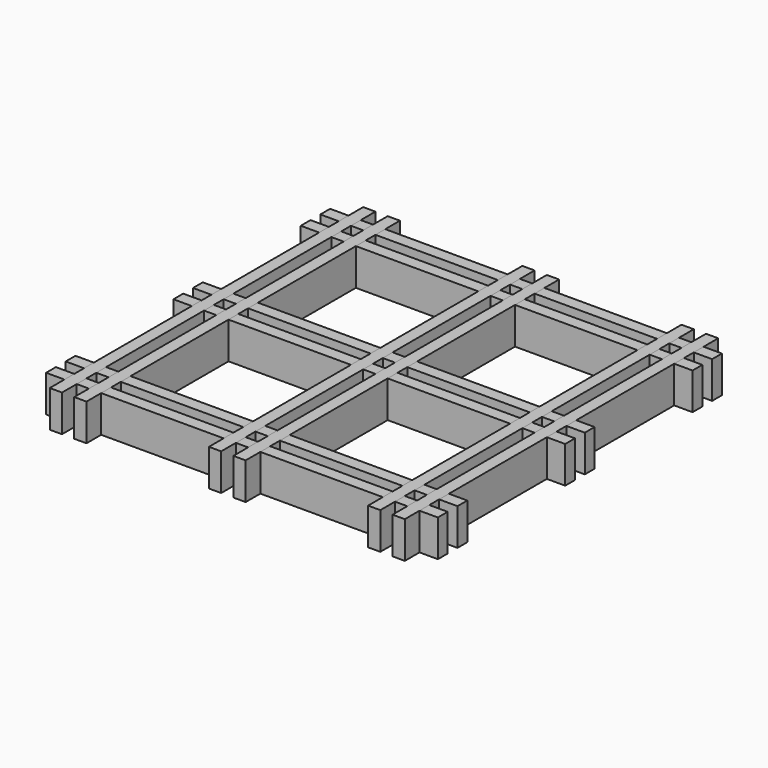
from build123d import *

# Parameters (mm, degrees)
F0_W     = 3.175
F0_H     = 101.6
F1_DEPTH = 9.525
F2_W     = 3.175
F2_H     = 4.7625
F3_DEPTH = 92.076
F4_W     = 101.6
F4_H     = 3.175
F5_DEPTH = 4.7625
F6_W     = 3.175
F6_H     = 3.175
F6_W_2   = 31.75
F6_W_3   = 4.7625
F7_DEPTH = 4.7625


with BuildPart() as f1:
    # F0 (on Top) → F1 (new body)
    with BuildSketch(Plane.XY):
        with Locations((1.5875, -50.8)):
            Rectangle(F0_W, F0_H)
    extrude(amount=F1_DEPTH)


with BuildPart() as f1b:
    # F0 (on Top) → F1, piece 2 (new body)
    with BuildSketch(Plane.XY):
        with Locations((7.9375, -50.8)):
            Rectangle(F0_W, F0_H)
    extrude(amount=F1_DEPTH)


with BuildPart() as f1c:
    # F0 (on Top) → F1, piece 3 (new body)
    with BuildSketch(Plane.XY):
        with Locations((42.8625, -50.8)):
            Rectangle(F0_W, F0_H)
    extrude(amount=F1_DEPTH)


with BuildPart() as f1d:
    # F0 (on Top) → F1, piece 4 (new body)
    with BuildSketch(Plane.XY):
        with Locations((49.2125, -50.8)):
            Rectangle(F0_W, F0_H)
    extrude(amount=F1_DEPTH)


with BuildPart() as f1e:
    # F0 (on Top) → F1, piece 5 (new body)
    with BuildSketch(Plane.XY):
        with Locations((84.1375, -50.8)):
            Rectangle(F0_W, F0_H)
    extrude(amount=F1_DEPTH)


with BuildPart() as f1f:
    # F0 (on Top) → F1, piece 6 (new body)
    with BuildSketch(Plane.XY):
        with Locations((90.4875, -50.8)):
            Rectangle(F0_W, F0_H)
    extrude(amount=F1_DEPTH)


with BuildPart() as f3_tool:
    # F2 (on face) → F3 (new body, through all)
    with BuildSketch(Plane.YZ.offset(92.075)):
        with Locations((-95.25, 2.38125)):
            Rectangle(F2_W, F2_H)
        with Locations((-47.625, 2.38125)):
            Rectangle(F2_W, F2_H)
        with Locations((-53.975, 2.38125)):
            Rectangle(F2_W, F2_H)
        with Locations((-6.35, 2.38125)):
            Rectangle(F2_W, F2_H)
        with Locations((-12.7, 2.38125)):
            Rectangle(F2_W, F2_H)
        with Locations((-88.9, 2.38125)):
            Rectangle(F2_W, F2_H)
    extrude(amount=-F3_DEPTH)


with BuildPart() as f1_1:
    add(f1.part)

    # F3: cut by f3_tool
    add(f3_tool.part, mode=Mode.SUBTRACT)


with BuildPart() as f1b_1:
    add(f1b.part)

    # F3: cut by f3_tool
    add(f3_tool.part, mode=Mode.SUBTRACT)


with BuildPart() as f1c_1:
    add(f1c.part)

    # F3: cut by f3_tool
    add(f3_tool.part, mode=Mode.SUBTRACT)


with BuildPart() as f1d_1:
    add(f1d.part)

    # F3: cut by f3_tool
    add(f3_tool.part, mode=Mode.SUBTRACT)


with BuildPart() as f1e_1:
    add(f1e.part)

    # F3: cut by f3_tool
    add(f3_tool.part, mode=Mode.SUBTRACT)


with BuildPart() as f1f_1:
    add(f1f.part)

    # F3: cut by f3_tool
    add(f3_tool.part, mode=Mode.SUBTRACT)


with BuildPart() as f5:
    # F4 (on Top) → F5 (new body, through all)
    with BuildSketch(Plane.XY):
        with Locations((46.0375, -6.35)):
            Rectangle(F4_W, F4_H)
    extrude(amount=F5_DEPTH)

    # F6 (on face) → F7, piece 6 (join, through all)
    with BuildSketch(Plane.XY.offset(4.7625)):
        with Locations((4.7625, -6.35)):
            Rectangle(F6_W, F6_H)
        with Locations((25.4, -6.35)):
            Rectangle(F6_W_2, F6_H)
        with Locations((94.45625, -6.35)):
            Rectangle(F6_W_3, F6_H)
        with Locations((-2.38125, -6.35)):
            Rectangle(F6_W_3, F6_H)
        with Locations((46.0375, -6.35)):
            Rectangle(F6_W, F6_H)
        with Locations((87.3125, -6.35)):
            Rectangle(F6_W, F6_H)
        with Locations((66.675, -6.35)):
            Rectangle(F6_W_2, F6_H)
    extrude(amount=F7_DEPTH)


with BuildPart() as f5b:
    # F4 (on Top) → F5, piece 2 (new body, through all)
    with BuildSketch(Plane.XY):
        with Locations((46.0375, -12.7)):
            Rectangle(F4_W, F4_H)
    extrude(amount=F5_DEPTH)

    # F6 (on face) → F7, piece 5 (join, through all)
    with BuildSketch(Plane.XY.offset(4.7625)):
        with Locations((4.7625, -12.7)):
            Rectangle(F6_W, F6_H)
        with Locations((25.4, -12.7)):
            Rectangle(F6_W_2, F6_H)
        with Locations((94.45625, -12.7)):
            Rectangle(F6_W_3, F6_H)
        with Locations((-2.38125, -12.7)):
            Rectangle(F6_W_3, F6_H)
        with Locations((46.0375, -12.7)):
            Rectangle(F6_W, F6_H)
        with Locations((87.3125, -12.7)):
            Rectangle(F6_W, F6_H)
        with Locations((66.675, -12.7)):
            Rectangle(F6_W_2, F6_H)
    extrude(amount=F7_DEPTH)


with BuildPart() as f5c:
    # F4 (on Top) → F5, piece 3 (new body, through all)
    with BuildSketch(Plane.XY):
        with Locations((46.0375, -95.25)):
            Rectangle(F4_W, F4_H)
    extrude(amount=F5_DEPTH)

    # F6 (on face) → F7 (join, through all)
    with BuildSketch(Plane.XY.offset(4.7625)):
        with Locations((4.7625, -95.25)):
            Rectangle(F6_W, F6_H)
        with Locations((25.4, -95.25)):
            Rectangle(F6_W_2, F6_H)
        with Locations((94.45625, -95.25)):
            Rectangle(F6_W_3, F6_H)
        with Locations((-2.38125, -95.25)):
            Rectangle(F6_W_3, F6_H)
        with Locations((46.0375, -95.25)):
            Rectangle(F6_W, F6_H)
        with Locations((87.3125, -95.25)):
            Rectangle(F6_W, F6_H)
        with Locations((66.675, -95.25)):
            Rectangle(F6_W_2, F6_H)
    extrude(amount=F7_DEPTH)


with BuildPart() as f5d:
    # F4 (on Top) → F5, piece 4 (new body, through all)
    with BuildSketch(Plane.XY):
        with Locations((46.0375, -47.625)):
            Rectangle(F4_W, F4_H)
    extrude(amount=F5_DEPTH)

    # F6 (on face) → F7, piece 4 (join, through all)
    with BuildSketch(Plane.XY.offset(4.7625)):
        with Locations((-2.38125, -47.625)):
            Rectangle(F6_W_3, F6_H)
        with Locations((4.7625, -47.625)):
            Rectangle(F6_W, F6_H)
        with Locations((25.4, -47.625)):
            Rectangle(F6_W_2, F6_H)
        with Locations((46.0375, -47.625)):
            Rectangle(F6_W, F6_H)
        with Locations((94.45625, -47.625)):
            Rectangle(F6_W_3, F6_H)
        with Locations((87.3125, -47.625)):
            Rectangle(F6_W, F6_H)
        with Locations((66.675, -47.625)):
            Rectangle(F6_W_2, F6_H)
    extrude(amount=F7_DEPTH)


with BuildPart() as f5e:
    # F4 (on Top) → F5, piece 5 (new body, through all)
    with BuildSketch(Plane.XY):
        with Locations((46.0375, -53.975)):
            Rectangle(F4_W, F4_H)
    extrude(amount=F5_DEPTH)

    # F6 (on face) → F7, piece 3 (join, through all)
    with BuildSketch(Plane.XY.offset(4.7625)):
        with Locations((-2.38125, -53.975)):
            Rectangle(F6_W_3, F6_H)
        with Locations((4.7625, -53.975)):
            Rectangle(F6_W, F6_H)
        with Locations((25.4, -53.975)):
            Rectangle(F6_W_2, F6_H)
        with Locations((46.0375, -53.975)):
            Rectangle(F6_W, F6_H)
        with Locations((87.3125, -53.975)):
            Rectangle(F6_W, F6_H)
        with Locations((94.45625, -53.975)):
            Rectangle(F6_W_3, F6_H)
        with Locations((66.675, -53.975)):
            Rectangle(F6_W_2, F6_H)
    extrude(amount=F7_DEPTH)


with BuildPart() as f5f:
    # F4 (on Top) → F5, piece 6 (new body, through all)
    with BuildSketch(Plane.XY):
        with Locations((46.0375, -88.9)):
            Rectangle(F4_W, F4_H)
    extrude(amount=F5_DEPTH)

    # F6 (on face) → F7, piece 2 (join, through all)
    with BuildSketch(Plane.XY.offset(4.7625)):
        with Locations((-2.38125, -88.9)):
            Rectangle(F6_W_3, F6_H)
        with Locations((4.7625, -88.9)):
            Rectangle(F6_W, F6_H)
        with Locations((25.4, -88.9)):
            Rectangle(F6_W_2, F6_H)
        with Locations((46.0375, -88.9)):
            Rectangle(F6_W, F6_H)
        with Locations((87.3125, -88.9)):
            Rectangle(F6_W, F6_H)
        with Locations((94.45625, -88.9)):
            Rectangle(F6_W_3, F6_H)
        with Locations((66.675, -88.9)):
            Rectangle(F6_W_2, F6_H)
    extrude(amount=F7_DEPTH)


solid = Compound([f1_1.part, f1b_1.part, f1c_1.part, f1d_1.part, f1e_1.part, f1f_1.part, f5.part, f5b.part, f5c.part, f5d.part, f5e.part, f5f.part])
